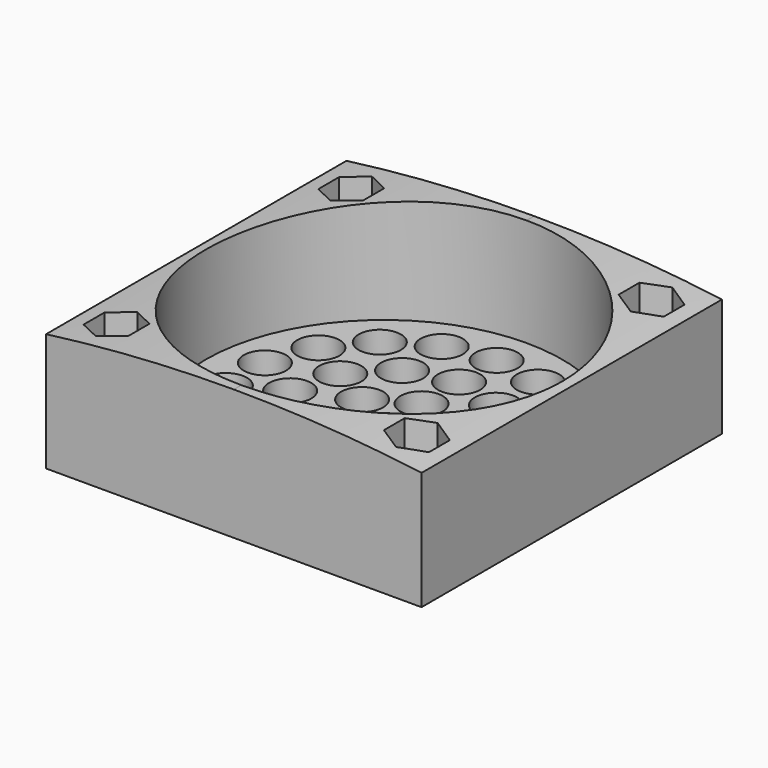
from build123d import *
from build123d import SkipClean  # not in build123d's __all__

# Parameters (mm, degrees)
F0_W     = 40
F0_H     = 40
F1_DEPTH = 13.918
F3_DEPTH = 25
F4_R     = 19
F5_DEPTH = 11.5
F7_DEPTH = 50
F8_R     = 2.25
F9_DEPTH = 25


with BuildPart() as f1:
    # F0 (on Top) → F1 (new body)
    with BuildSketch(Plane.XY):
        Rectangle(F0_W, F0_H)
    extrude(amount=F1_DEPTH)

    # F2 (on face) → F3 (cut)
    with BuildSketch(Plane.XY.offset(13.918)):
        Polygon((-13.6, 17.0143593539), (-16, 18.4), (-18.4, 17.0143593539), (-18.4, 14.2430780618), (-16, 12.8574374158), (-13.6, 14.2430780618), align=None)
        Polygon((13.6, 17.0143593539), (13.6, 14.2430780618), (16, 12.8574374158), (18.4, 14.2430780618), (18.4, 17.0143593539), (16, 18.4), align=None)
        Polygon((-13.6, -17.0143593539), (-13.6, -14.2430780618), (-16, -12.8574374158), (-18.4, -14.2430780618), (-18.4, -17.0143593539), (-16, -18.4), align=None)
        Polygon((18.4, -14.2430780618), (16, -12.8574374158), (13.6, -14.2430780618), (13.6, -17.0143593539), (16, -18.4), (18.4, -17.0143593539), align=None)
    extrude(amount=-F3_DEPTH, mode=Mode.SUBTRACT)

    # F4 (on face) → F5 (cut)
    with BuildSketch(Plane.XY.offset(13.918)):
        Circle(F4_R)
    extrude(amount=-F5_DEPTH, mode=Mode.SUBTRACT)

    # F6 (on face) → F7 (cut)
    with BuildSketch(Plane(origin=(0, 20, 0), x_dir=(-1, 0, 0), z_dir=(0, 1, 0))):
        with BuildLine():
            ThreePointArc((-20, 12.5999645093), (-10.021691693, 13.5881341343), (0, 13.918))
            Line((0, 13.918), (-20, 13.918))
            Line((-20, 13.918), (-20, 12.5999645093))
        make_face()
        with BuildLine():
            ThreePointArc((0, 13.918), (10.021691693, 13.5881341343), (20, 12.5999645093))
            Line((20, 12.5999645093), (20, 13.918))
            Line((20, 13.918), (0, 13.918))
        make_face()
    with SkipClean():  # cleaning this boolean's faces spoils the solid; the shape is the same uncleaned
        extrude(amount=-F7_DEPTH, mode=Mode.SUBTRACT)

    # F8 (on face) → F9 (cut)
    with BuildSketch(Plane(origin=(0, 0, 0), x_dir=(1, 0, 0), z_dir=(0, 0, -1))):
        Circle(F8_R)
        with Locations((0, 5)):
            Circle(F8_R)
        with Locations((-4.3301270189, 2.5)):
            Circle(F8_R)
        with Locations((-4.3301270189, -2.5)):
            Circle(F8_R)
        with Locations((0, -5)):
            Circle(F8_R)
        with Locations((4.3301270189, -2.5)):
            Circle(F8_R)
        with Locations((4.3301270189, 2.5)):
            Circle(F8_R)
        with Locations((0, 10)):
            Circle(F8_R)
        with Locations((0, 15)):
            Circle(F8_R)
        with Locations((-5.1303021499, 14.0953893118)):
            Circle(F8_R)
        with Locations((-9.6418141453, 11.4906666468)):
            Circle(F8_R)
        with Locations((-12.9903810568, 7.5)):
            Circle(F8_R)
        with Locations((-14.7721162952, 2.604722665)):
            Circle(F8_R)
        with Locations((-14.7721162952, -2.604722665)):
            Circle(F8_R)
        with Locations((-12.9903810568, -7.5)):
            Circle(F8_R)
        with Locations((-9.6418141453, -11.4906666468)):
            Circle(F8_R)
        with Locations((-5.1303021499, -14.0953893118)):
            Circle(F8_R)
        with Locations((0, -15)):
            Circle(F8_R)
        with Locations((5.1303021499, -14.0953893118)):
            Circle(F8_R)
        with Locations((9.6418141453, -11.4906666468)):
            Circle(F8_R)
        with Locations((12.9903810568, -7.5)):
            Circle(F8_R)
        with Locations((14.7721162952, -2.604722665)):
            Circle(F8_R)
        with Locations((14.7721162952, 2.604722665)):
            Circle(F8_R)
        with Locations((12.9903810568, 7.5)):
            Circle(F8_R)
        with Locations((9.6418141453, 11.4906666468)):
            Circle(F8_R)
        with Locations((5.1303021499, 14.0953893118)):
            Circle(F8_R)
        with Locations((-5, 8.6602540378)):
            Circle(F8_R)
        with Locations((-8.6602540378, 5)):
            Circle(F8_R)
        with Locations((-10, 0)):
            Circle(F8_R)
        with Locations((-8.6602540378, -5)):
            Circle(F8_R)
        with Locations((-5, -8.6602540378)):
            Circle(F8_R)
        with Locations((0, -10)):
            Circle(F8_R)
        with Locations((5, -8.6602540378)):
            Circle(F8_R)
        with Locations((8.6602540378, -5)):
            Circle(F8_R)
        with Locations((10, 0)):
            Circle(F8_R)
        with Locations((8.6602540378, 5)):
            Circle(F8_R)
        with Locations((5, 8.6602540378)):
            Circle(F8_R)
    with SkipClean():  # cleaning this boolean's faces spoils the solid; the shape is the same uncleaned
        extrude(amount=-F9_DEPTH, mode=Mode.SUBTRACT)


solid = f1.part
